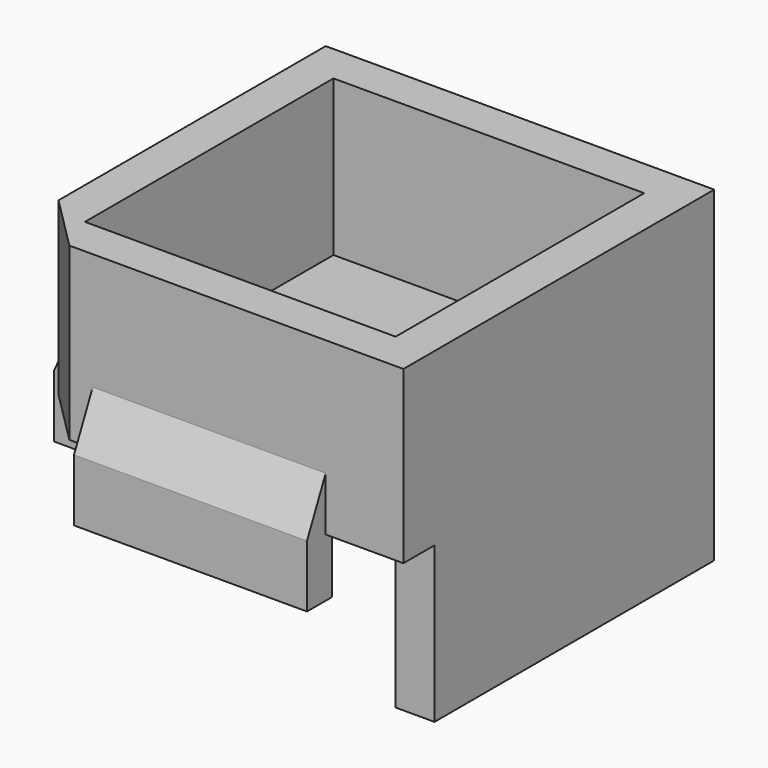
from build123d import *

# Parameters (mm, degrees)
F1_DEPTH     = 20
F0_W         = 39.9660819769
F0_H         = 39.9660819769
F2_DEPTH     = 2
F4_DEPTH     = 20
F5_W         = 29.9660819769
F5_H         = 7.5
F6_DEPTH     = 3
F7_T4_DEPTH  = 66.2397385768
F8_W         = 29.9660819769
F8_H         = 7.5
F9_DEPTH     = 3
F10_T4_DEPTH = 66.2397385768
F11_DEPTH    = 1
F12_DEPTH    = 1
F13_SIZE     = 7


# Not quite as in the source:
# - a fillet or chamfer that OpenCascade refuses, or shapes differently, is made with other operations: its cross-section is extruded or revolved along the edge and cut away or added


with BuildPart() as f1:
    # F0 (on Top) → F1 (new body)
    with BuildSketch(Plane.XY):
        Polygon((24.9830409884, -24.9830409884), (24.9830409884, 19.9830409884), (19.9830409884, 19.9830409884), (19.9830409884, -19.9830409884), (-19.9830409884, -19.9830409884), (-19.9830409884, -24.9830409884), align=None)
        Polygon((24.9830409884, 24.9830409884), (-24.9830409884, 24.9830409884), (-24.9830409884, -24.9830409884), (-19.9830409884, -24.9830409884), (-19.9830409884, -19.9830409884), (-19.9830409884, 19.9830409884), (19.9830409884, 19.9830409884), (24.9830409884, 19.9830409884), align=None)
    extrude(amount=F1_DEPTH)

    # F0 (on Top) → F2 (join)
    with BuildSketch(Plane.XY):
        Polygon((24.9830409884, 24.9830409884), (-24.9830409884, 24.9830409884), (-24.9830409884, -24.9830409884), (-19.9830409884, -24.9830409884), (-19.9830409884, -19.9830409884), (-19.9830409884, 19.9830409884), (19.9830409884, 19.9830409884), (24.9830409884, 19.9830409884), align=None)
        Rectangle(F0_W, F0_H)
        Polygon((24.9830409884, -24.9830409884), (24.9830409884, 19.9830409884), (19.9830409884, 19.9830409884), (19.9830409884, -19.9830409884), (-19.9830409884, -19.9830409884), (-19.9830409884, -24.9830409884), align=None)
    extrude(amount=-F2_DEPTH)

    # F3 (on face) → F4 (join)
    with BuildSketch(Plane(origin=(0, 0, -2), x_dir=(1, 0, 0), z_dir=(0, 0, -1))):
        Polygon((24.9830409884, -24.9830409884), (24.9830409884, 19.9830409884), (19.9830409884, 19.9830409884), (19.9830409884, -19.9830409884), (-19.9830409884, -19.9830409884), (-19.9830409884, -24.9830409884), align=None)
    extrude(amount=F4_DEPTH)

    # F5 (on face) → F6 (join)
    with BuildSketch(Plane(origin=(-24.9830409884, 0, 0), x_dir=(0, -1, 0), z_dir=(-1, 0, 0))):
        with Locations((0, 1.75)):
            Rectangle(F5_W, F5_H)
        with Locations((0, -5.75)):
            Rectangle(F5_W, F5_H)
    extrude(amount=F6_DEPTH)

    # F7: chamfer of 7 x 3.2641536071 on 1 edges, made by hand


with BuildPart() as f7_tool2:
    # F7_s3 → F7_t4 (new body)
    with BuildSketch(Plane.XZ.offset(33.1198692884)):
        Polygon((-24.7188873814, 5.5), (-27.9830409884, -1.5), (-27.9830409884, 5.5), align=None)
    extrude(amount=-F7_T4_DEPTH)

    split(bisect_by=Plane.YZ.offset(-24.9830409884), keep=Keep.BOTTOM)


with BuildPart() as f1_1:
    add(f1.part)

    # F7_t1: cut F7_tool2
    add(f7_tool2.part, mode=Mode.SUBTRACT)

    # F8 (on face) → F9 (join)
    with BuildSketch(Plane.XZ.offset(24.9830409884)):
        with Locations((0, 1.75)):
            Rectangle(F8_W, F8_H)
        with Locations((0, -5.75)):
            Rectangle(F8_W, F8_H)
    extrude(amount=F9_DEPTH)

    # F10: chamfer of 7 x 3.2641536071 on 1 edges, made by hand


with BuildPart() as f10_tool2:
    # F10_s3 → F10_t4 (new body)
    with BuildSketch(Plane.YZ.offset(33.1198692884)):
        Polygon((-24.7188873814, 5.5), (-27.9830409884, -1.5), (-27.9830409884, 5.5), align=None)
    extrude(amount=-F10_T4_DEPTH)

    split(bisect_by=Plane.XZ.offset(24.9830409884), keep=Keep.TOP)


with BuildPart() as f1_2:
    add(f1_1.part)

    # F10_t1: cut F10_tool2
    add(f10_tool2.part, mode=Mode.SUBTRACT)

    # F11 (add): a face of the model
    f11_faces = [f1_2.faces().sort_by_distance(p)[0] for p in [
        (0, -24.9830409884, -5.75),
    ]]
    extrude(f11_faces, amount=F11_DEPTH)

    # F12 (add): a face of the model
    f12_faces = [f1_2.faces().sort_by_distance(p)[0] for p in [
        (-24.9830409884, 0, -5.75),
    ]]
    extrude(f12_faces, amount=F12_DEPTH)

    # F13
    f13_edges = [f1_2.edges().sort_by_distance(p)[0] for p in [
        (-24.983041, -24.983041, 9),
    ]]
    chamfer(f13_edges, length=F13_SIZE)


solid = f1_2.part
